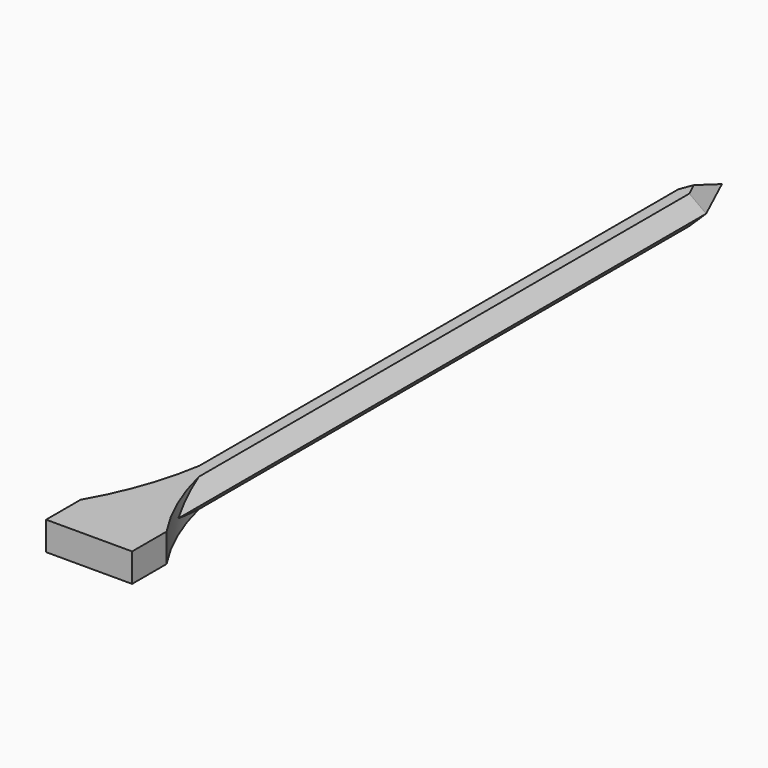
from build123d import *

# Parameters (mm, degrees)
F1_DEPTH = 2.5
F2_SIZE  = 2.49999
F4_DEPTH = 2.5


# Not quite as in the source:
# - a fillet or chamfer is up to 0.001 mm smaller than in the source, because OpenCascade refuses the exact size


with BuildPart() as f1:
    # F0 (on Top) → F1 (new body, symmetric)
    with BuildSketch(Plane.XY):
        Polygon((-3.1822135206, 54.0976710618), (-3.1822135206, -76.2216448784), (3.7883522455, -76.2216448784), (3.7883522455, 54.0976710618), (0, 62.2805096209), align=None)
    extrude(amount=F1_DEPTH, both=True)

    # F2 (size 2.5 in the source; OpenCascade refuses exactly that, so slightly less here)
    f2_edges = [f1.edges().sort_by_distance(p)[0] for p in [
        (-1.591107, 58.18909, -2.5),
        (-3.182214, -11.061987, -2.5),
        (0.303069, -76.221645, -2.5),
        (3.788352, -11.061987, -2.5),
        (1.894176, 58.18909, -2.5),
        (-1.591107, 58.18909, 2.5),
        (-3.182214, -11.061987, 2.5),
        (0.303069, -76.221645, 2.5),
        (3.788352, -11.061987, 2.5),
        (1.894176, 58.18909, 2.5),
    ]]
    chamfer(f2_edges, length=F2_SIZE)

    # F3 (on Top) → F4 (join, symmetric)
    with BuildSketch(Plane.XY):
        with BuildLine():
            Line((-7.067034021, -69.0257325768), (-7.067034021, -76.5438452363))
            Line((-7.067034021, -76.5438452363), (7.9692080617, -76.5438452363))
            Line((7.9692080617, -76.5438452363), (7.9692080617, -69.0257325768))
            ThreePointArc((7.9692080617, -69.0257325768), (2.0355302464, -56.380771616), (0, -42.5619371235))
            ThreePointArc((0, -42.5619371235), (-1.7971813817, -56.2575152388), (-7.067034021, -69.0257325768))
        make_face()
    extrude(amount=F4_DEPTH, both=True)


solid = f1.part
